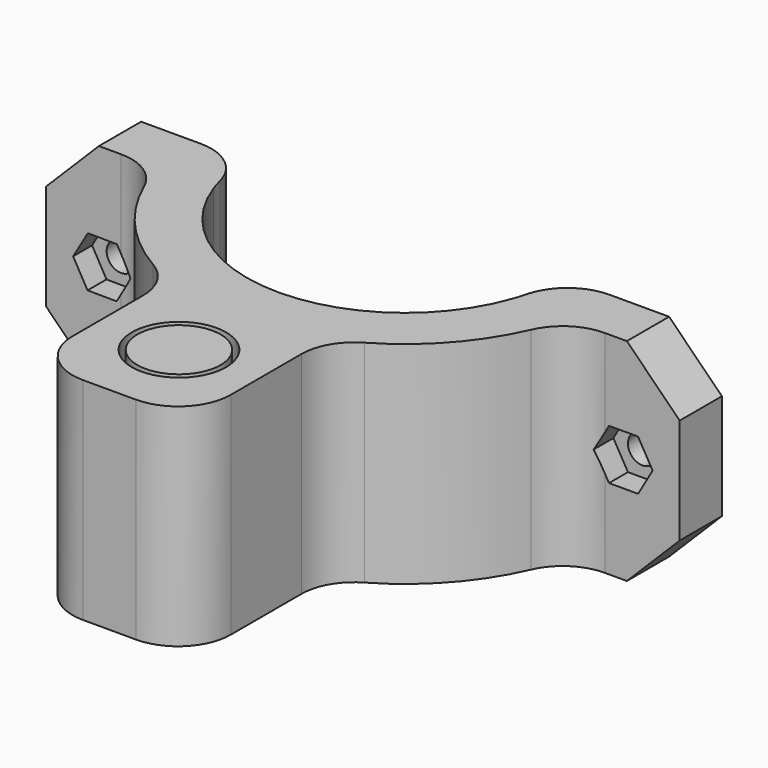
from build123d import *

# Parameters (mm, degrees)
F1_DEPTH     = 50.8
F3_DEPTH     = 12.7
F4_SIZE      = 12.7
F5_R         = 11.35
F5_R_2       = 10
F6_DEPTH     = 44.45
F7_T1_DEPTH  = 50.8
F7_T6_DEPTH  = 73.3295570728
F7_T11_DEPTH = 73.3295570728
F7_T16_DEPTH = 73.3295570728
F7_T21_DEPTH = 73.3295570728
F7_T23_DEPTH = 114.3
F8_R         = 3.5
F9_DEPTH     = 50.801
F10_W        = 183.8439181447
F10_H        = 157.3934331536
F11_DEPTH    = 63.5
F12_R        = 12.7
F13_R        = 3.5
F13_W        = 17.6573731005
F13_H        = 18.0775066838
F14_DEPTH    = 7


# Not quite as in the source:
# - a fillet or chamfer that OpenCascade refuses, or shapes differently, is made with other operations: its cross-section is extruded or revolved along the edge and cut away or added


with BuildPart() as f1:
    # F0 (on Top) → F1 (new body)
    with BuildSketch(Plane.XY):
        with BuildLine():
            ThreePointArc((-35.9210244843, 12.7), (0, 38.1), (35.9210244843, 12.7))
            Line((35.9210244843, 12.7), (49.1868884968, 12.7))
            ThreePointArc((49.1868884968, 12.7), (0, 50.8), (-49.1868884968, 12.7))
            Line((-49.1868884968, 12.7), (-35.9210244843, 12.7))
        make_face()
        with BuildLine():
            ThreePointArc((-49.1868884968, -12.7), (-50.8, 0), (-49.1868884968, 12.7))
            Line((-49.1868884968, 12.7), (-76.2, 12.7))
            Line((-76.2, 12.7), (-76.2, -12.7))
            Line((-76.2, -12.7), (-49.1868884968, -12.7))
        make_face()
        with BuildLine():
            ThreePointArc((-35.9210244843, -12.7), (-38.1, 0), (-35.9210244843, 12.7))
            Line((-35.9210244843, 12.7), (-49.1868884968, 12.7))
            ThreePointArc((-49.1868884968, 12.7), (-50.8, 0), (-49.1868884968, -12.7))
            Line((-49.1868884968, -12.7), (-35.9210244843, -12.7))
        make_face()
        with BuildLine():
            ThreePointArc((35.9210244843, 12.7), (37.5513051228, 6.4427853895), (38.1, 0))
            ThreePointArc((38.1, 0), (37.5513051228, -6.4427853895), (35.9210244843, -12.7))
            Line((35.9210244843, -12.7), (49.1868884968, -12.7))
            ThreePointArc((49.1868884968, -12.7), (50.3951085704, -6.4010180581), (50.8, 0))
            ThreePointArc((50.8, 0), (50.3951085704, 6.4010180581), (49.1868884968, 12.7))
            Line((49.1868884968, 12.7), (35.9210244843, 12.7))
        make_face()
        with BuildLine():
            Line((76.2, 12.7), (49.1868884968, 12.7))
            ThreePointArc((49.1868884968, 12.7), (50.3951085704, 6.4010180581), (50.8, 0))
            ThreePointArc((50.8, 0), (50.3951085704, -6.4010180581), (49.1868884968, -12.7))
            Line((49.1868884968, -12.7), (76.2, -12.7))
            Line((76.2, -12.7), (76.2, 12.7))
        make_face()
        with BuildLine():
            ThreePointArc((-19.05, -32.9955678842), (-29.2989914869, -24.3552683798), (-35.9210244843, -12.7))
            Line((-35.9210244843, -12.7), (-49.1868884968, -12.7))
            ThreePointArc((-49.1868884968, -12.7), (-38.2071387235, -33.479165918), (-19.05, -47.0928603931))
            Line((-19.05, -47.0928603931), (-19.05, -32.9955678842))
        make_face()
        with BuildLine():
            Line((49.1868884968, -12.7), (35.9210244843, -12.7))
            ThreePointArc((35.9210244843, -12.7), (29.2989914869, -24.3552683798), (19.05, -32.9955678842))
            Line((19.05, -32.9955678842), (19.05, -47.0928603931))
            ThreePointArc((19.05, -47.0928603931), (38.2071387235, -33.479165918), (49.1868884968, -12.7))
        make_face()
        with BuildLine():
            Line((19.05, -47.0928603931), (19.05, -32.9955678842))
            ThreePointArc((19.05, -32.9955678842), (0, -38.1), (-19.05, -32.9955678842))
            Line((-19.05, -32.9955678842), (-19.05, -47.0928603931))
            ThreePointArc((-19.05, -47.0928603931), (0, -50.8), (19.05, -47.0928603931))
        make_face()
        with BuildLine():
            Line((19.05, -88.9), (19.05, -47.0928603931))
            ThreePointArc((19.05, -47.0928603931), (0, -50.8), (-19.05, -47.0928603931))
            Line((-19.05, -47.0928603931), (-19.05, -88.9))
            Line((-19.05, -88.9), (19.05, -88.9))
        make_face()
    extrude(amount=F1_DEPTH)

    # F2 (on face) → F3 (cut)
    with BuildSketch(Plane.XZ.offset(12.7)):
        Polygon((-55.6935602012, 25.3597094836), (-59.1586096141, 31.4419321502), (-66.1584936613, 31.4822226666), (-69.6933282956, 25.4402905164), (-66.2282788827, 19.3580678498), (-59.2283948355, 19.3177773334), align=None)
        Polygon((59.1938884968, 31.4621778265), (55.6938884968, 25.4), (59.1938884968, 19.3378221735), (66.1938884968, 19.3378221735), (69.6938884968, 25.4), (66.1938884968, 31.4621778265), align=None)
    extrude(amount=-F3_DEPTH, mode=Mode.SUBTRACT)

    # F4
    f4_edges = [f1.edges().sort_by_distance(p)[0] for p in [
        (-76.2, 0, 50.8),
        (-76.2, 0, 0),
        (76.2, 0, 50.8),
        (76.2, 0, 0),
    ]]
    chamfer(f4_edges, length=F4_SIZE)

    # F5 (on face) → F6 (cut)
    with BuildSketch(Plane.XY.offset(50.8)):
        with Locations((0, -67.9964301965)):
            Circle(F5_R)
        with Locations((0, -67.9964301965)):
            Circle(F5_R_2, mode=Mode.SUBTRACT)
    extrude(amount=-F6_DEPTH, mode=Mode.SUBTRACT)

    # F7: fillet of radius 12.7 on 8 edges, made by hand

    # F7_s2 → F7_t1 (join)
    with BuildSketch(Plane.XY):
        with BuildLine():
            ThreePointArc((-25.4, -43.9940905122), (-20.7514773719, -48.6426131403), (-19.05, -54.9926131403))
            Line((-19.05, -54.9926131403), (-19.05, -47.0928603931))
            ThreePointArc((-19.05, -47.0928603931), (-22.2789411484, -45.6540116672), (-25.4, -43.9940905122))
        make_face()
        with BuildLine():
            ThreePointArc((25.4, -43.9940905122), (20.7514773719, -48.6426131403), (19.05, -54.9926131403))
            Line((19.05, -54.9926131403), (19.05, -47.0928603931))
            ThreePointArc((19.05, -47.0928603931), (22.2789411484, -45.6540116672), (25.4, -43.9940905122))
        make_face()
    extrude(amount=F7_T1_DEPTH)


with BuildPart() as f7_tool4:
    # F7_s5 → F7_t6 (new body)
    with BuildSketch(Plane.XY):
        with BuildLine():
            ThreePointArc((58.1987113259, -12.7), (51.2426348456, -14.774417663), (46.5589690608, -20.32))
            ThreePointArc((46.5589690608, -20.32), (48.0243002017, -16.562203662), (49.1868884968, -12.7))
            Line((49.1868884968, -12.7), (58.1987113259, -12.7))
        make_face()
    extrude(amount=F7_T6_DEPTH)

    split(bisect_by=Plane(origin=(52.7689390007, 0, 30.4661611369), x_dir=(0, 1, 0), z_dir=(-0.8660254038, 0, -0.5)), keep=Keep.TOP)


with BuildPart() as f1_1:
    add(f1.part)

    # F7_t3: union F7_tool4
    add(f7_tool4.part)


with BuildPart() as f7_tool9:
    # F7_s10 → F7_t11 (new body)
    with BuildSketch(Plane.XY.offset(-22.5295570728)):
        with BuildLine():
            ThreePointArc((58.1987113259, -12.7), (51.2426348456, -14.774417663), (46.5589690608, -20.32))
            ThreePointArc((46.5589690608, -20.32), (48.0243002017, -16.562203662), (49.1868884968, -12.7))
            Line((49.1868884968, -12.7), (58.1987113259, -12.7))
        make_face()
    extrude(amount=F7_T11_DEPTH)

    split(bisect_by=Plane(origin=(30.7718937446, 0, -17.7661611369), x_dir=(0, 1, 0), z_dir=(-0.8660254038, 0, 0.5)), keep=Keep.TOP)


with BuildPart() as f1_2:
    add(f1_1.part)

    # F7_t8: union F7_tool9
    add(f7_tool9.part)


with BuildPart() as f7_tool14:
    # F7_s15 → F7_t16 (new body)
    with BuildSketch(Plane.XY):
        with BuildLine():
            ThreePointArc((-58.1987113259, -12.7), (-51.2426348456, -14.774417663), (-46.5589690608, -20.32))
            ThreePointArc((-46.5589690608, -20.32), (-48.0243002017, -16.562203662), (-49.1868884968, -12.7))
            Line((-49.1868884968, -12.7), (-58.1987113259, -12.7))
        make_face()
    extrude(amount=F7_T16_DEPTH)

    split(bisect_by=Plane(origin=(-52.5449689068, 0, 30.7414534512), x_dir=(0, 1, 0), z_dir=(0.8631331643, 0, -0.5049763763)), keep=Keep.TOP)


with BuildPart() as f1_3:
    add(f1_2.part)

    # F7_t13: union F7_tool14
    add(f7_tool14.part)


with BuildPart() as f7_tool19:
    # F7_s20 → F7_t21 (new body)
    with BuildSketch(Plane.XY.offset(-22.5295570728)):
        with BuildLine():
            ThreePointArc((-58.1987113259, -12.7), (-51.2426348456, -14.774417663), (-46.5589690608, -20.32))
            ThreePointArc((-46.5589690608, -20.32), (-48.0243002017, -16.562203662), (-49.1868884968, -12.7))
            Line((-49.1868884968, -12.7), (-58.1987113259, -12.7))
        make_face()
    extrude(amount=F7_T21_DEPTH)

    split(bisect_by=Plane(origin=(-31.1394890128, 0, -17.7402035465), x_dir=(0, 1, 0), z_dir=(0.8688889524, 0, 0.495007059)), keep=Keep.TOP)


with BuildPart() as f1_4:
    add(f1_3.part)

    # F7_t18: union F7_tool19
    add(f7_tool19.part)

    # F7_s24 → F7_t23 (cut)
    with BuildSketch(Plane.XY.offset(-31.75)):
        with BuildLine():
            ThreePointArc((-6.35, -88.9), (-15.3302561211, -85.1802561211), (-19.05, -76.2))
            Line((-19.05, -76.2), (-19.05, -88.9))
            Line((-19.05, -88.9), (-6.35, -88.9))
        make_face()
        with BuildLine():
            ThreePointArc((19.05, -76.2), (15.3302561211, -85.1802561211), (6.35, -88.9))
            Line((6.35, -88.9), (19.05, -88.9))
            Line((19.05, -88.9), (19.05, -76.2))
        make_face()
    extrude(amount=F7_T23_DEPTH, mode=Mode.SUBTRACT)

    # F8 (on face) → F9 (cut, through all)
    with BuildSketch(Plane.XZ):
        with Locations((-62.6585516377, 25.4402905164)):
            Circle(F8_R)
        with Locations((62.6938884968, 25.4402905164)):
            Circle(F8_R)
    extrude(amount=-F9_DEPTH, mode=Mode.SUBTRACT)

    # F10 (on Front) → F11 (cut)
    with BuildSketch(Plane.XZ):
        with Locations((-6.0164444149, -2.5229565799)):
            Rectangle(F10_W, F10_H)
    extrude(amount=-F11_DEPTH, mode=Mode.SUBTRACT)

    # F12
    f12_edges = [f1_4.edges().sort_by_distance(p)[0] for p in [
        (38.1, 0, 25.4),
        (-38.1, 0, 25.4),
    ]]
    fillet(f12_edges, radius=F12_R)

    # F13 (on face) → F14 (join)
    with BuildSketch(Plane(origin=(0, 0, 0), x_dir=(-1, 0, 0), z_dir=(0, 1, 0))):
        Polygon((-55.6938884968, 25.4), (-59.1938884968, 31.4621778265), (-66.1938884968, 31.4621778265), (-69.6938884968, 25.4), (-66.1938884968, 19.3378221735), (-59.1938884968, 19.3378221735), align=None)
        with Locations((-62.6938884968, 25.4)):
            Circle(F13_R, mode=Mode.SUBTRACT)
        with Locations((63.3883532137, 24.6192668565)):
            Rectangle(F13_W, F13_H)
        with Locations((62.6936761559, 25.3597094836)):
            Circle(F13_R, mode=Mode.SUBTRACT)
    extrude(amount=-F14_DEPTH)


solid = f1_4.part
